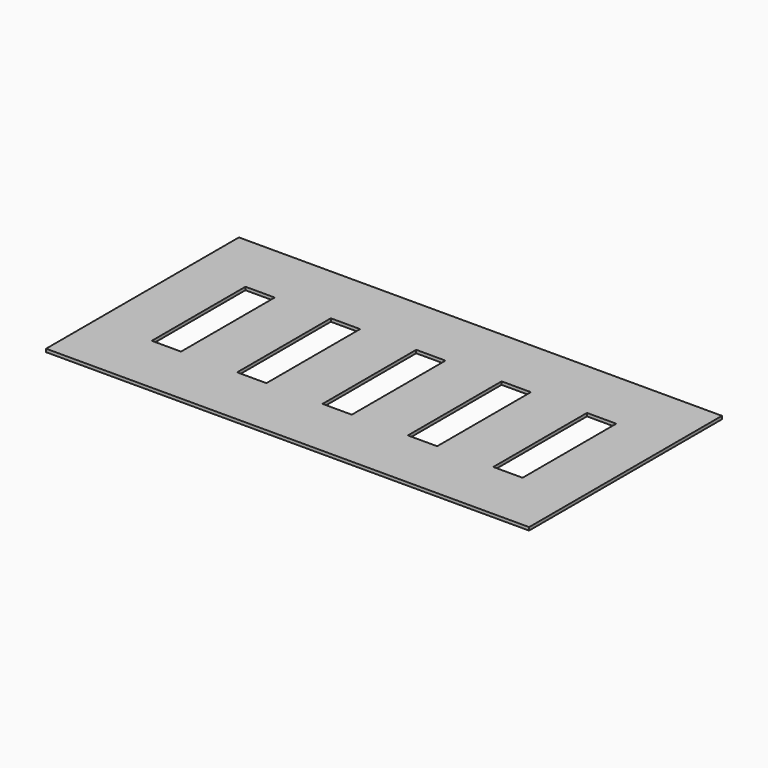
from build123d import *

# Parameters (mm, degrees)
F1_DEPTH = 3.175


# Not quite as in the source:
# - a length typed as a fraction of an inch, garbled in the dataset ("3 / 203.2 mm" for 3/8 in), is restored


with BuildPart() as f1:
    # F0 (on Top) → F1 (new body)
    with BuildSketch(Plane.XY):
        Polygon((247.5, 123.5), (-247.5, 123.5), (-247.5, 0), (-190, 0), (-190, 60), (-160, 60), (-160, 0), (-102.5, 0), (-102.5, 60), (-72.5, 60), (-72.5, 0), (-15, 0), (-15, 60), (15, 60), (15, 0), (72.5, 0), (72.5, 60), (102.5, 60), (102.5, 0), (160, 0), (160, 60), (190, 60), (190, 0), (247.5, 0), align=None)
        Polygon((-190, 0), (-247.5, 0), (-247.5, -123.5), (247.5, -123.5), (247.5, 0), (190, 0), (190, -60), (160, -60), (160, 0), (102.5, 0), (102.5, -60), (72.5, -60), (72.5, 0), (15, 0), (15, -60), (-15, -60), (-15, 0), (-72.5, 0), (-72.5, -60), (-102.5, -60), (-102.5, 0), (-160, 0), (-160, -60), (-190, -60), align=None)
    extrude(amount=-F1_DEPTH)


solid = f1.part
